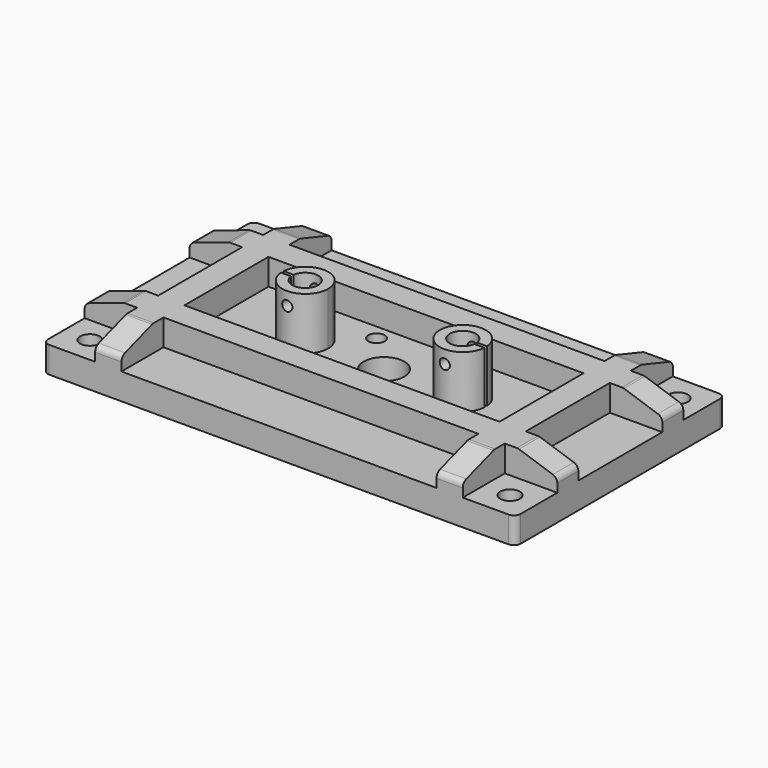
from build123d import *

# Parameters (mm, degrees)
F0_W           = 228.6
F0_H           = 127
F0_R           = 4.7625
F0_R_2         = 4.0005
F0_R_3         = 6.2865
F0_R_4         = 9.8425
F1_DEPTH       = 12.7
F2_R           = 11.1125
F2_R_2         = 6.2865
F3_DEPTH       = 25.4
F4_W           = 23.2800319791
F4_H           = 1.5875
F5_DEPTH       = 25.4
F6_W           = 12.7
F6_H           = 127
F7_DEPTH       = 12.7
F8_W           = 228.6
F8_H           = 12.7
F9_DEPTH       = 12.7
F10_R          = 3.175
F11_SIZE2      = 6.35
F11_SIZE       = 19.05
F12_R          = 3.175
F13_R          = 2.4765
F14_DEPTH      = 25.4
F14_DEPTH_BACK = 25.4


with BuildPart() as f1:
    # F0 (on Top) → F1 (new body)
    with BuildSketch(Plane.XY):
        Rectangle(F0_W, F0_H)
        with Locations((-101.6, -50.8)):
            Circle(F0_R, mode=Mode.SUBTRACT)
        with Locations((-17.9451, -17.9451)):
            Circle(F0_R_2, mode=Mode.SUBTRACT)
        with Locations((101.6, -50.8)):
            Circle(F0_R, mode=Mode.SUBTRACT)
        with Locations((17.9451, -17.9451)):
            Circle(F0_R_2, mode=Mode.SUBTRACT)
        with Locations((-38.1, 0)):
            Circle(F0_R_3, mode=Mode.SUBTRACT)
        with Locations((-17.9451, 17.9451)):
            Circle(F0_R_2, mode=Mode.SUBTRACT)
        with Locations((-101.6, 50.8)):
            Circle(F0_R, mode=Mode.SUBTRACT)
        Circle(F0_R_4, mode=Mode.SUBTRACT)
        with Locations((38.1, 0)):
            Circle(F0_R_3, mode=Mode.SUBTRACT)
        with Locations((17.9451, 17.9451)):
            Circle(F0_R_2, mode=Mode.SUBTRACT)
        with Locations((101.6, 50.8)):
            Circle(F0_R, mode=Mode.SUBTRACT)
    extrude(amount=F1_DEPTH)

    # F2 (on face) → F3 (join)
    with BuildSketch(Plane.XY.offset(12.7)):
        with Locations((-38.1, 0)):
            Circle(F2_R)
        with Locations((-38.1, 0)):
            Circle(F2_R_2, mode=Mode.SUBTRACT)
        with Locations((38.1, 0)):
            Circle(F2_R)
        with Locations((38.1, 0)):
            Circle(F2_R_2, mode=Mode.SUBTRACT)
    extrude(amount=F3_DEPTH)

    # F4 (on face) → F5 (cut, through all)
    with BuildSketch(Plane.XY.offset(38.1)):
        with Locations((53.7348873913, 0)):
            Rectangle(F4_W, F4_H)
        with BuildLine():
            Line((-37.5724840105, -0.79375), (-37.5724840105, 0.79375))
            Line((-37.5724840105, 0.79375), (-44.3361881937, 0.79375))
            ThreePointArc((-44.3361881937, 0.79375), (-44.3865, 0), (-44.3361881937, -0.79375))
            Line((-44.3361881937, -0.79375), (-37.5724840105, -0.79375))
        make_face()
        with BuildLine():
            ThreePointArc((-44.3361881937, -0.79375), (-44.3865, 0), (-44.3361881937, 0.79375))
            Line((-44.3361881937, 0.79375), (-49.1841155347, 0.79375))
            ThreePointArc((-49.1841155347, 0.79375), (-49.2125, 0), (-49.1841155347, -0.79375))
            Line((-49.1841155347, -0.79375), (-44.3361881937, -0.79375))
        make_face()
        with BuildLine():
            ThreePointArc((-49.1841155347, -0.79375), (-49.2125, 0), (-49.1841155347, 0.79375))
            Line((-49.1841155347, 0.79375), (-60.8525159895, 0.79375))
            Line((-60.8525159895, 0.79375), (-60.8525159895, -0.79375))
            Line((-60.8525159895, -0.79375), (-49.1841155347, -0.79375))
        make_face()
    extrude(amount=-F5_DEPTH, mode=Mode.SUBTRACT)

    # F6 (on face) → F7 (join)
    with BuildSketch(Plane.XY.offset(12.7)):
        with Locations((-82.55, 0)):
            Rectangle(F6_W, F6_H)
        with Locations((82.55, 0)):
            Rectangle(F6_W, F6_H)
    extrude(amount=F7_DEPTH)

    # F8 (on face) → F9 (join)
    with BuildSketch(Plane.XY.offset(12.7)):
        with Locations((0, -31.75)):
            Rectangle(F8_W, F8_H)
        with Locations((0, 31.75)):
            Rectangle(F8_W, F8_H)
    extrude(amount=F9_DEPTH)

    # F10
    f10_edges = [f1.edges().sort_by_distance(p)[0] for p in [
        (-114.3, -63.5, 6.35),
        (114.3, -63.5, 6.35),
        (-114.3, 63.5, 6.35),
        (114.3, 63.5, 6.35),
    ]]
    fillet(f10_edges, radius=F10_R)

    # F11
    f11_edges = [f1.edges().sort_by_distance(p)[0] for p in [
        (-114.3, 31.75, 25.4),
        (-114.3, -31.75, 25.4),
        (114.3, -31.75, 25.4),
        (114.3, 31.75, 25.4),
        (-82.55, -63.5, 25.4),
        (82.55, -63.5, 25.4),
        (82.55, 63.5, 25.4),
        (-82.55, 63.5, 25.4),
    ]]
    f11_side = f1.faces().sort_by_distance((78.81509, 50.8, 25.4))[0]
    chamfer(f11_edges, length=F11_SIZE, length2=F11_SIZE2, reference=f11_side)

    # F12
    f12_edges = [f1.edges().sort_by_distance(p)[0] for p in [
        (-114.3, -31.75, 19.05),
        (-114.3, 31.75, 19.05),
        (-95.25, 31.75, 25.4),
        (-95.25, -31.75, 25.4),
        (95.25, -31.75, 25.4),
        (114.3, -31.75, 19.05),
        (114.3, 31.75, 19.05),
        (95.25, 31.75, 25.4),
        (-82.55, -63.5, 19.05),
        (82.55, -63.5, 19.05),
        (82.55, -44.45, 25.4),
        (-82.55, -44.45, 25.4),
        (-82.55, 44.45, 25.4),
        (-82.55, 63.5, 19.05),
        (82.55, 44.45, 25.4),
        (82.55, 63.5, 19.05),
    ]]
    fillet(f12_edges, radius=F12_R)

    # F13 (on Front) → F14 (cut, two sides)
    with BuildSketch(Plane.XZ) as f14_sk:
        with Locations((-38.1, 31.75)):
            Circle(F13_R)
        with Locations((38.1, 31.75)):
            Circle(F13_R)
    extrude(amount=-F14_DEPTH, mode=Mode.SUBTRACT)
    extrude(f14_sk.sketch, amount=F14_DEPTH_BACK, mode=Mode.SUBTRACT)


solid = f1.part
